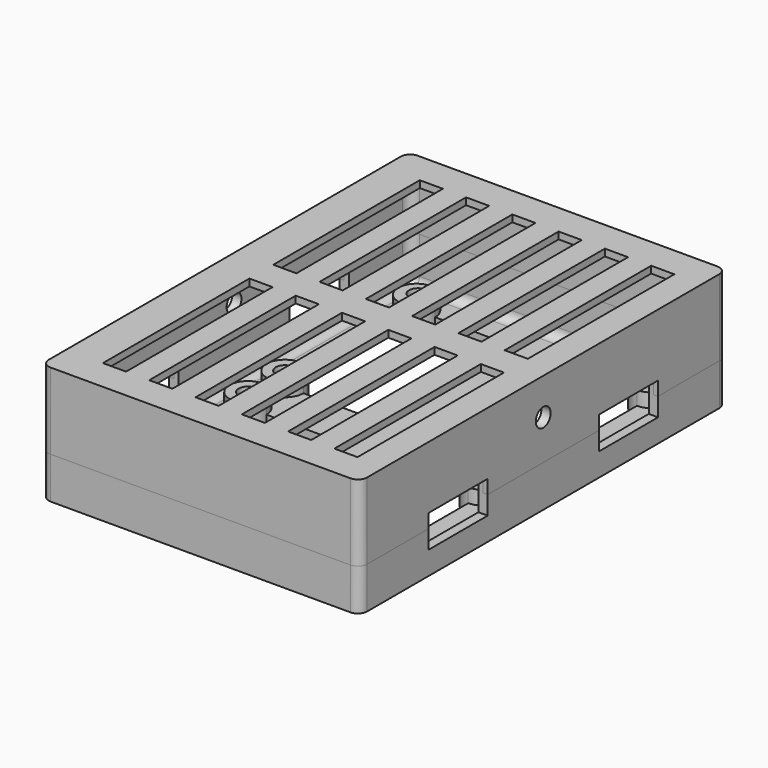
from build123d import *

# Parameters (mm, degrees)
F1_DEPTH       = 2
F2_DEPTH       = 5
F3_DEPTH       = 12
F5_DEPTH       = 3
F7_W           = 5
F7_H           = 39.56
F8_DEPTH       = 1.5
F9_DEPTH       = 15
F10_DEPTH      = 12
F11_W          = 16
F11_H          = 7
F11_R          = 2
F12_DEPTH      = 40
F12_DEPTH_BACK = 40
F13_R          = 2
F13_2_R        = 2


with BuildPart() as f1:
    # F0 (on Top) → F1 (new body)
    with BuildSketch(Plane.XY):
        Polygon((-34.4, 26.56), (-34.4, -26.56), (34.4, -26.56), (34.4, 26.56), (34.4, 72.56), (-34.4, 72.56), align=None)
        Polygon((32.4, -24.56), (-32.4, -24.56), (-32.4, 24.56), (-32.4, 70.56), (32.4, 70.56), (32.4, 24.56), align=None, mode=Mode.SUBTRACT)
        Polygon((-32.4, 24.56), (-32.4, -24.56), (32.4, -24.56), (32.4, 24.56), (32.4, 70.56), (-32.4, 70.56), align=None)
        with BuildLine():
            ThreePointArc((-25.4, 22), (-22.5715728753, 20.8284271247), (-21.4, 18))
            Line((-21.4, 18), (-5, 18))
            Line((-5, 18), (-5, -17.56))
            Line((-5, -17.56), (-21.4, -17.56))
            ThreePointArc((-21.4, -17.56), (-28.2284271247, -20.3884271247), (-25.4, -13.56))
            Line((-25.4, -13.56), (-25.4, 14))
            ThreePointArc((-25.4, 14), (-29.4, 18), (-25.4, 22))
        make_face(mode=Mode.SUBTRACT)
        with BuildLine():
            ThreePointArc((25.4, 22), (28.2284271247, 20.8284271247), (29.4, 18))
            ThreePointArc((29.4, 18), (28.2284271247, 15.1715728753), (25.4, 14))
            Line((25.4, 14), (25.4, -13.56))
            ThreePointArc((25.4, -13.56), (28.2284271247, -14.7315728753), (29.4, -17.56))
            ThreePointArc((29.4, -17.56), (25.4, -21.56), (21.4, -17.56))
            Line((21.4, -17.56), (5, -17.56))
            Line((5, -17.56), (5, 18))
            Line((5, 18), (21.4, 18))
            ThreePointArc((21.4, 18), (22.5715728753, 20.8284271247), (25.4, 22))
        make_face(mode=Mode.SUBTRACT)
        with BuildLine():
            ThreePointArc((-21.4, 28), (-22.5715728753, 25.1715728753), (-25.4, 24))
            ThreePointArc((-25.4, 24), (-29.4, 28), (-25.4, 32))
            Line((-25.4, 32), (-25.4, 59.56))
            ThreePointArc((-25.4, 59.56), (-28.2284271247, 66.3884271247), (-21.4, 63.56))
            Line((-21.4, 63.56), (-5, 63.56))
            Line((-5, 63.56), (-5, 28))
            Line((-5, 28), (-21.4, 28))
        make_face(mode=Mode.SUBTRACT)
        with BuildLine():
            ThreePointArc((29.4, 28), (28.2284271247, 25.1715728753), (25.4, 24))
            ThreePointArc((25.4, 24), (22.5715728753, 25.1715728753), (21.4, 28))
            Line((21.4, 28), (5, 28))
            Line((5, 28), (5, 63.56))
            Line((5, 63.56), (21.4, 63.56))
            ThreePointArc((21.4, 63.56), (25.4, 67.56), (29.4, 63.56))
            ThreePointArc((29.4, 63.56), (28.2284271247, 60.7315728753), (25.4, 59.56))
            Line((25.4, 59.56), (25.4, 32))
            ThreePointArc((25.4, 32), (28.2284271247, 30.8284271247), (29.4, 28))
        make_face(mode=Mode.SUBTRACT)
    extrude(amount=F1_DEPTH)

    # F0 (on Top) → F2 (join)
    with BuildSketch(Plane.XY):
        with BuildLine():
            Line((-23.4, 18), (-21.4, 18))
            ThreePointArc((-21.4, 18), (-22.5715728753, 20.8284271247), (-25.4, 22))
            Line((-25.4, 22), (-25.4, 20))
            ThreePointArc((-25.4, 20), (-23.9857864376, 19.4142135624), (-23.4, 18))
        make_face()
        with BuildLine():
            Line((-25.4, 20), (-25.4, 22))
            ThreePointArc((-25.4, 22), (-29.4, 18), (-25.4, 14))
            Line((-25.4, 14), (-25.4, 16))
            ThreePointArc((-25.4, 16), (-27.4, 18), (-25.4, 20))
        make_face()
        with BuildLine():
            ThreePointArc((-25.4, 14), (-22.5715728753, 15.1715728753), (-21.4, 18))
            Line((-21.4, 18), (-23.4, 18))
            ThreePointArc((-23.4, 18), (-23.9857864376, 16.5857864376), (-25.4, 16))
            Line((-25.4, 16), (-25.4, 14))
        make_face()
        with BuildLine():
            Line((25.4, 20), (25.4, 22))
            ThreePointArc((25.4, 22), (22.5715728753, 20.8284271247), (21.4, 18))
            Line((21.4, 18), (23.4, 18))
            ThreePointArc((23.4, 18), (23.9857864376, 19.4142135624), (25.4, 20))
        make_face()
        with BuildLine():
            ThreePointArc((21.4, 18), (22.5715728753, 15.1715728753), (25.4, 14))
            Line((25.4, 14), (25.4, 16))
            ThreePointArc((25.4, 16), (23.9857864376, 16.5857864376), (23.4, 18))
            Line((23.4, 18), (21.4, 18))
        make_face()
        with BuildLine():
            ThreePointArc((25.4, 14), (28.2284271247, 15.1715728753), (29.4, 18))
            ThreePointArc((29.4, 18), (28.2284271247, 20.8284271247), (25.4, 22))
            Line((25.4, 22), (25.4, 20))
            ThreePointArc((25.4, 20), (26.8142135624, 19.4142135624), (27.4, 18))
            ThreePointArc((27.4, 18), (26.8142135624, 16.5857864376), (25.4, 16))
            Line((25.4, 16), (25.4, 14))
        make_face()
        with BuildLine():
            Line((25.4, -16), (25.4, -13.56))
            ThreePointArc((25.4, -13.56), (22.5715728753, -14.7315728753), (21.4, -17.56))
            Line((21.4, -17.56), (23.4490002563, -17.56))
            ThreePointArc((23.4490002563, -17.56), (24.1510004003, -16.4379500648), (25.4, -16))
        make_face()
        with BuildLine():
            ThreePointArc((29.4, -17.56), (28.2284271247, -14.7315728753), (25.4, -13.56))
            Line((25.4, -13.56), (25.4, -16))
            ThreePointArc((25.4, -16), (26.8142135624, -16.5857864376), (27.4, -18))
            ThreePointArc((27.4, -18), (25.1786399849, -19.9877121884), (23.4490002563, -17.56))
            Line((23.4490002563, -17.56), (21.4, -17.56))
            ThreePointArc((21.4, -17.56), (25.4, -21.56), (29.4, -17.56))
        make_face()
        with BuildLine():
            ThreePointArc((-21.4, -17.56), (-22.5715728753, -14.7315728753), (-25.4, -13.56))
            Line((-25.4, -13.56), (-25.4, -16))
            ThreePointArc((-25.4, -16), (-24.1510004003, -16.4379500648), (-23.4490002563, -17.56))
            Line((-23.4490002563, -17.56), (-21.4, -17.56))
        make_face()
        with BuildLine():
            Line((-25.4, -16), (-25.4, -13.56))
            ThreePointArc((-25.4, -13.56), (-28.2284271247, -20.3884271247), (-21.4, -17.56))
            Line((-21.4, -17.56), (-23.4490002563, -17.56))
            ThreePointArc((-23.4490002563, -17.56), (-23.4122878116, -17.7786399849), (-23.4, -18))
            ThreePointArc((-23.4, -18), (-26.8142135624, -19.4142135624), (-25.4, -16))
        make_face()
        with BuildLine():
            ThreePointArc((-25.4, 32), (-29.4, 28), (-25.4, 24))
            ThreePointArc((-25.4, 24), (-22.5715728753, 25.1715728753), (-21.4, 28))
            ThreePointArc((-21.4, 28), (-22.5715728753, 30.8284271247), (-25.4, 32))
        make_face()
        with BuildLine():
            ThreePointArc((-23.4, 28), (-23.9857864376, 26.5857864376), (-25.4, 26))
            ThreePointArc((-25.4, 26), (-26.8142135624, 29.4142135624), (-23.4, 28))
        make_face(mode=Mode.SUBTRACT)
        with BuildLine():
            ThreePointArc((-21.4, 63.56), (-28.2284271247, 66.3884271247), (-25.4, 59.56))
            Line((-25.4, 59.56), (-25.4, 62))
            ThreePointArc((-25.4, 62), (-26.8142135624, 65.4142135624), (-23.4, 64))
            ThreePointArc((-23.4, 64), (-23.4122878116, 63.7786399849), (-23.4490002563, 63.56))
            Line((-23.4490002563, 63.56), (-21.4, 63.56))
        make_face()
        with BuildLine():
            Line((-25.4, 62), (-25.4, 59.56))
            ThreePointArc((-25.4, 59.56), (-22.5715728753, 60.7315728753), (-21.4, 63.56))
            Line((-21.4, 63.56), (-23.4490002563, 63.56))
            ThreePointArc((-23.4490002563, 63.56), (-24.1510004003, 62.4379500648), (-25.4, 62))
        make_face()
        with BuildLine():
            ThreePointArc((21.4, 63.56), (22.5715728753, 60.7315728753), (25.4, 59.56))
            Line((25.4, 59.56), (25.4, 62))
            ThreePointArc((25.4, 62), (24.1510004003, 62.4379500648), (23.4490002563, 63.56))
            Line((23.4490002563, 63.56), (21.4, 63.56))
        make_face()
        with BuildLine():
            Line((25.4, 62), (25.4, 59.56))
            ThreePointArc((25.4, 59.56), (28.2284271247, 60.7315728753), (29.4, 63.56))
            ThreePointArc((29.4, 63.56), (25.4, 67.56), (21.4, 63.56))
            Line((21.4, 63.56), (23.4490002563, 63.56))
            ThreePointArc((23.4490002563, 63.56), (25.1786399849, 65.9877121884), (27.4, 64))
            ThreePointArc((27.4, 64), (26.8142135624, 62.5857864376), (25.4, 62))
        make_face()
        with BuildLine():
            ThreePointArc((25.4, 32), (22.5715728753, 30.8284271247), (21.4, 28))
            Line((21.4, 28), (23.4, 28))
            ThreePointArc((23.4, 28), (23.9857864376, 29.4142135624), (25.4, 30))
            Line((25.4, 30), (25.4, 32))
        make_face()
        with BuildLine():
            ThreePointArc((21.4, 28), (22.5715728753, 25.1715728753), (25.4, 24))
            Line((25.4, 24), (25.4, 26))
            ThreePointArc((25.4, 26), (23.9857864376, 26.5857864376), (23.4, 28))
            Line((23.4, 28), (21.4, 28))
        make_face()
        with BuildLine():
            Line((25.4, 26), (25.4, 24))
            ThreePointArc((25.4, 24), (28.2284271247, 25.1715728753), (29.4, 28))
            ThreePointArc((29.4, 28), (28.2284271247, 30.8284271247), (25.4, 32))
            Line((25.4, 32), (25.4, 30))
            ThreePointArc((25.4, 30), (26.8142135624, 29.4142135624), (27.4, 28))
            ThreePointArc((27.4, 28), (26.8142135624, 26.5857864376), (25.4, 26))
        make_face()
    extrude(amount=F2_DEPTH)

    # F0 (on Top) → F3 (join)
    with BuildSketch(Plane.XY):
        Polygon((-34.4, 26.56), (-34.4, -26.56), (34.4, -26.56), (34.4, 26.56), (34.4, 72.56), (-34.4, 72.56), align=None)
        Polygon((32.4, -24.56), (-32.4, -24.56), (-32.4, 24.56), (-32.4, 70.56), (32.4, 70.56), (32.4, 24.56), align=None, mode=Mode.SUBTRACT)
    extrude(amount=F3_DEPTH)

    # F4 (on face) → F5 (cut)
    with BuildSketch(Plane.XY.offset(12)):
        Polygon((-34.4, 26.56), (-34.4, -26.56), (34.4, -26.56), (34.4, 26.56), (34.4, 72.56), (-34.4, 72.56), align=None)
        Polygon((33.4, -25.2946496815), (-33.4, -25.2946496815), (-33.4, 20.7053503185), (-33.4, 25.2946496815), (-33.4, 71.2946496815), (33.4, 71.2946496815), (33.4, 25.2946496815), (33.4, 20.7053503185), align=None, mode=Mode.SUBTRACT)
    extrude(amount=-F5_DEPTH, mode=Mode.SUBTRACT)


with BuildPart() as f8:
    # F7 (on offset) → F8 (new body)
    with BuildSketch(Plane.XY.offset(24)):
        Polygon((-34.4, 72.56), (-34.4, 26.56), (-34.4, 19.44), (-34.4, -26.56), (34.4, -26.56), (34.4, 19.44), (34.4, 26.56), (34.4, 72.56), align=None)
        Polygon((33.4, 71.56), (33.4, 23.78), (33.4, -25.2946496815), (33.4, -25.56), (-33.4, -25.56), (-33.4, -25.2946496815), (-33.4, 71.56), align=None, mode=Mode.SUBTRACT)
        Polygon((33.4, -25.2946496815), (33.4, 23.78), (33.4, 71.56), (-33.4, 71.56), (-33.4, -25.2946496815), (-33.4, -25.56), (33.4, -25.56), align=None)
        Polygon((32.4, -24.56), (-32.4, -24.56), (-32.4, 24.56), (-32.4, 70.56), (32.4, 70.56), (32.4, 21), align=None, mode=Mode.SUBTRACT)
        Polygon((-32.4, 24.56), (-32.4, -24.56), (32.4, -24.56), (32.4, 21), (32.4, 70.56), (-32.4, 70.56), align=None)
        with Locations((-24, 0)):
            Rectangle(F7_W, F7_H, mode=Mode.SUBTRACT)
        with Locations((-14, 0)):
            Rectangle(F7_W, F7_H, mode=Mode.SUBTRACT)
        with Locations((-4, 0)):
            Rectangle(F7_W, F7_H, mode=Mode.SUBTRACT)
        with Locations((6, 0)):
            Rectangle(F7_W, F7_H, mode=Mode.SUBTRACT)
        with Locations((16, 0)):
            Rectangle(F7_W, F7_H, mode=Mode.SUBTRACT)
        with Locations((26, 0)):
            Rectangle(F7_W, F7_H, mode=Mode.SUBTRACT)
        with Locations((-24, 46)):
            Rectangle(F7_W, F7_H, mode=Mode.SUBTRACT)
        with Locations((-14, 46)):
            Rectangle(F7_W, F7_H, mode=Mode.SUBTRACT)
        with Locations((-4, 46)):
            Rectangle(F7_W, F7_H, mode=Mode.SUBTRACT)
        with Locations((6, 46)):
            Rectangle(F7_W, F7_H, mode=Mode.SUBTRACT)
        with Locations((16, 46)):
            Rectangle(F7_W, F7_H, mode=Mode.SUBTRACT)
        with Locations((26, 46)):
            Rectangle(F7_W, F7_H, mode=Mode.SUBTRACT)
    extrude(amount=F8_DEPTH)

    # F7 (on offset) → F9 (join)
    with BuildSketch(Plane.XY.offset(24)):
        Polygon((-34.4, 72.56), (-34.4, 26.56), (-34.4, 19.44), (-34.4, -26.56), (34.4, -26.56), (34.4, 19.44), (34.4, 26.56), (34.4, 72.56), align=None)
        Polygon((33.4, 71.56), (33.4, 23.78), (33.4, -25.2946496815), (33.4, -25.56), (-33.4, -25.56), (-33.4, -25.2946496815), (-33.4, 71.56), align=None, mode=Mode.SUBTRACT)
    extrude(amount=-F9_DEPTH)

    # F7 (on offset) → F10 (join)
    with BuildSketch(Plane.XY.offset(24)):
        Polygon((33.4, -25.2946496815), (33.4, 23.78), (33.4, 71.56), (-33.4, 71.56), (-33.4, -25.2946496815), (-33.4, -25.56), (33.4, -25.56), align=None)
        Polygon((32.4, -24.56), (-32.4, -24.56), (-32.4, 24.56), (-32.4, 70.56), (32.4, 70.56), (32.4, 21), align=None, mode=Mode.SUBTRACT)
    extrude(amount=-F10_DEPTH)


with BuildPart() as f12_tool:
    # F11 (on Right) → F12 (new body, two sides)
    with BuildSketch(Plane.YZ) as f12_sk:
        with Locations((0, 8.5)):
            Rectangle(F11_W, F11_H)
        with Locations((46, 8.5)):
            Rectangle(F11_W, F11_H)
        with Locations((23, 17.6025740802)):
            Circle(F11_R)
    extrude(amount=-F12_DEPTH)
    extrude(f12_sk.sketch, amount=F12_DEPTH_BACK)


with BuildPart() as f1_1:
    add(f1.part)

    # F12: cut by f12_tool
    add(f12_tool.part, mode=Mode.SUBTRACT)

    # F13
    f13_edges = [f1_1.edges().sort_by_distance(p)[0] for p in [
        (0, 70.56, 2),
        (-32.4, 23, 2),
        (32.4, 23, 2),
        (0, -24.56, 2),
        (34.4, -26.56, 4.5),
        (-34.4, -26.56, 4.5),
        (-34.4, 72.56, 4.5),
        (34.4, 72.56, 4.5),
        (-32.4, 70.56, 7),
        (32.4, 70.56, 7),
        (-32.4, -24.56, 7),
        (32.4, -24.56, 7),
    ]]
    fillet(f13_edges, radius=F13_R)


with BuildPart() as f8_1:
    add(f8.part)

    # F12: cut by f12_tool
    add(f12_tool.part, mode=Mode.SUBTRACT)

    # F13#2
    f13_2_edges = [f8_1.edges().sort_by_distance(p)[0] for p in [
        (34.4, 72.56, 17.25),
        (-34.4, 72.56, 17.25),
        (-34.4, -26.56, 17.25),
        (34.4, -26.56, 17.25),
        (0, -24.56, 24),
        (32.4, -24.56, 18),
        (-32.4, -24.56, 18),
        (32.4, 23, 24),
        (0, 70.56, 24),
        (32.4, 70.56, 18),
        (-32.4, 23, 24),
        (-32.4, 70.56, 18),
    ]]
    fillet(f13_2_edges, radius=F13_2_R)


solid = Compound([f1_1.part, f8_1.part])
